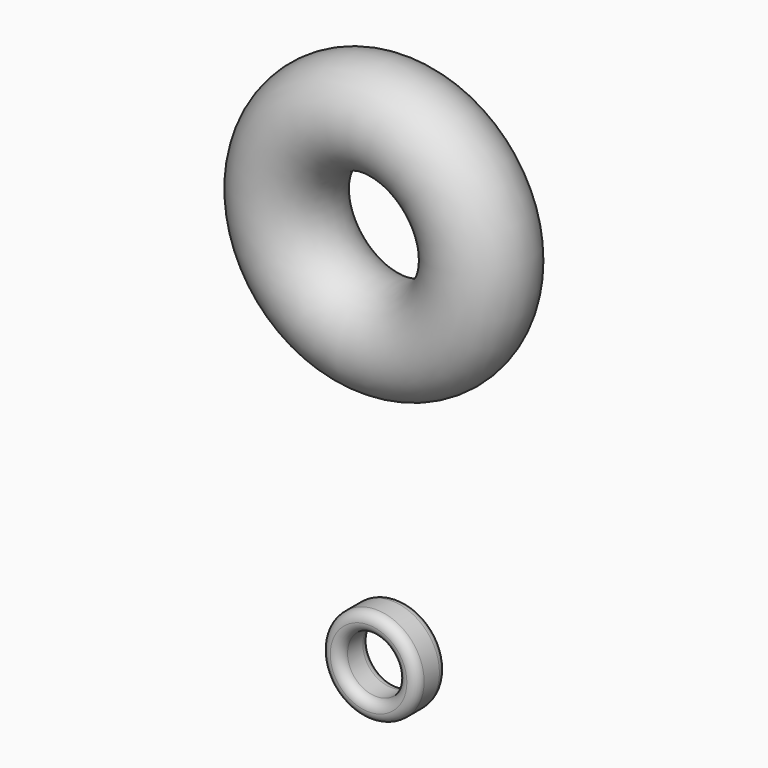
from build123d import *

# Parameters (mm, degrees)
F3_R     = 12.5000003539
F3_R_2   = 7.5
F4_DEPTH = 5
F5_R     = 2.49999


# Not quite as in the source:
# - a fillet or chamfer is up to 0.001 mm smaller than in the source, because OpenCascade refuses the exact size


with BuildPart() as f1:
    # F0 (on Top) → F1 (revolve)
    with BuildSketch(Plane.XY):
        with BuildLine():
            ThreePointArc((12.7, 0), (25.4, -12.7), (38.1, 0))
            ThreePointArc((38.1, 0), (25.4, 12.7), (12.7, 0))
        make_face()
    revolve(axis=Axis((0, 0, 0), (0, 1, 0)))


with BuildPart() as f1_1:
    # F2: moved
    add(f1.part.moved(Location((0, 0, 100))))


with BuildPart() as f4:
    # F3 (on Front) → F4 (new body, symmetric)
    with BuildSketch(Plane.XZ):
        Circle(F3_R)
        Circle(F3_R_2, mode=Mode.SUBTRACT)
    extrude(amount=F4_DEPTH, both=True)

    # F5 (radius 2.5 in the source; OpenCascade refuses exactly that, so slightly less here)
    f5_edges = [f4.edges().sort_by_distance(p)[0] for p in [
        (-12.5, -5, 0),
        (-12.5, 5, 0),
        (-7.5, -5, 0),
        (-7.5, 5, 0),
    ]]
    fillet(f5_edges, radius=F5_R)


solid = Compound([f1_1.part, f4.part])
